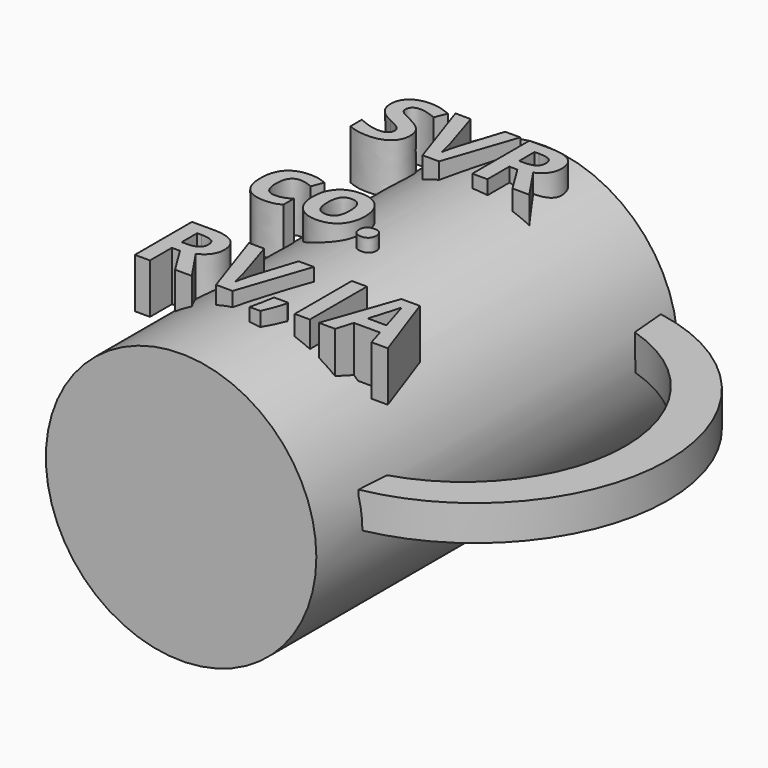
from build123d import *

# Parameters (mm, degrees)
F0_R         = 38.0185509889
F1_DEPTH     = 127
F2_R         = 30.8458248883
F3_DEPTH     = 123.952
F5_DEPTH     = 9.906
F7_START     = 27.686
F6_TEXT_SIZE = 28.0904919944
F7_DEPTH     = 13.97


# Not quite as in the source:
# - Text() gives the source's letters only with a copy of the font that has no kerning and outlines rounded to 1/6400 em; it was checked with that copy


with BuildPart() as f1:
    # F0 (on Front) → F1 (new body)
    with BuildSketch(Plane.XZ):
        Circle(F0_R)
    extrude(amount=F1_DEPTH)

    # F2 (on Front) → F3 (cut)
    with BuildSketch(Plane.XZ):
        Circle(F2_R)
    extrude(amount=F3_DEPTH, mode=Mode.SUBTRACT)

    # F4 (on Top) → F5 (join)
    with BuildSketch(Plane.XY):
        with BuildLine():
            ThreePointArc((37.6974865794, -14.7125702351), (69.9035243941, -58.2395670936), (37.6974865794, -101.766563952))
            Line((37.6974865794, -101.766563952), (37.0913892984, -110.9975129366))
            ThreePointArc((37.0913892984, -110.9975129366), (81.4264053178, -57.6046901423), (36.8155390024, -4.4421302155))
            Line((36.8155390024, -4.4421302155), (37.6974865794, -14.7125702351))
        make_face()
    extrude(amount=F5_DEPTH)

    # F6 (on Top) → F7 (join)
    with BuildSketch(Plane.XY.offset(F7_START)):
        with Locations((-35.3947281837, -25.7533360273)):
            Text('SVR', F6_TEXT_SIZE, font='Open Sans', font_style=FontStyle.BOLD, text_align=(TextAlign.LEFT, TextAlign.BOTTOM))
        with Locations((-35.3947281837, -63.9564051396)):
            Text('co.', F6_TEXT_SIZE, font='Open Sans', font_style=FontStyle.BOLD, text_align=(TextAlign.LEFT, TextAlign.BOTTOM))
        with Locations((-35.3947281837, -102.159474252)):
            Text('RV,IA', F6_TEXT_SIZE, font='Open Sans', font_style=FontStyle.BOLD, text_align=(TextAlign.LEFT, TextAlign.BOTTOM))
    extrude(amount=F7_DEPTH)


solid = f1.part
